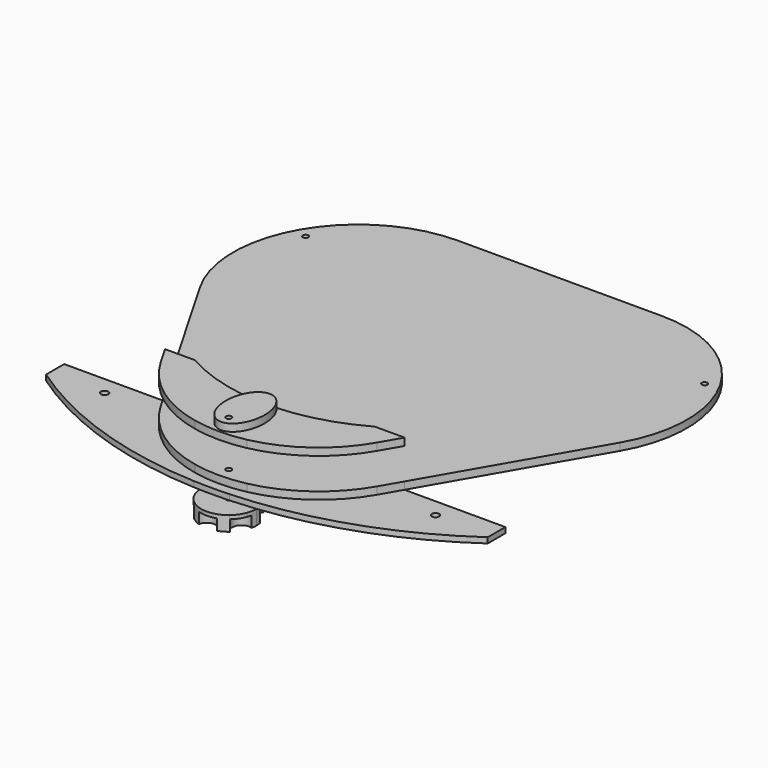
from build123d import *

# Parameters (mm, degrees)
F0_R     = 1.5
F1_DEPTH = 4
F0_R_2   = 2
F2_DEPTH = 3
F3_START = -10
F3_DEPTH = 8
F4_R     = 1.5
F5_DEPTH = 6
F6_START = 21
F6_DEPTH = 4
F7_R     = 1.5
F8_DEPTH = 4


with BuildPart() as f1:
    # F0 (on Top) → F1 (new body)
    with BuildSketch(Plane.XY):
        with BuildLine():
            ThreePointArc((14.9999983029, -125.2980828285), (-2.6585899749, -110.535565822), (-14.0575894796, -130.5310767839))
            ThreePointArc((-14.0575894796, -130.5310767839), (-1.8826e-06, -132), (14.0575857957, -130.5310775623))
            ThreePointArc((14.0575857957, -130.5310775623), (14.7625152359, -127.9566715151), (14.9999983029, -125.2980828285))
        make_face()
        with Locations((-1.6971e-06, -125.2980828285)):
            Circle(F0_R, mode=Mode.SUBTRACT)
        with BuildLine():
            Line((-48.9863926684, -87.1798906476), (-65.1367205046, -87.1798906476))
            Line((-65.1367205046, -87.1798906476), (-58.8897274573, -98))
            ThreePointArc((-58.8897274573, -98), (-39.9361427939, -119.0373009762), (-14.0575894796, -130.5310767839))
            ThreePointArc((-14.0575894796, -130.5310767839), (-2.6585899749, -110.535565822), (14.9999983029, -125.2980828285))
            ThreePointArc((14.9999983029, -125.2980828285), (14.7625152359, -127.9566715151), (14.0575857957, -130.5310775623))
            ThreePointArc((14.0575857957, -130.5310775623), (39.9361412701, -119.0373020819), (58.8897274573, -98))
            Line((58.8897274573, -98), (65.1367205046, -87.1798906476))
            Line((65.1367205046, -87.1798906476), (48.9863926684, -87.1798906476))
            ThreePointArc((48.9863926684, -87.1798906476), (0, -100), (-48.9863926684, -87.1798906476))
        make_face()
        with BuildLine():
            Line((-114.3153532995, -2), (-86.6025397374, -50.0000011103))
            ThreePointArc((-86.6025397374, -50.0000011103), (-86.6025407137, 49.9999994193), (-5.89e-08, 100))
            Line((-5.89e-08, 100), (-55.4256258422, 100))
            ThreePointArc((-55.4256258422, 100), (-114.3153532995, 66), (-114.3153532995, -2))
        make_face()
        with Locations((-108.5113219264, 62.649042884)):
            Circle(F0_R, mode=Mode.SUBTRACT)
        with BuildLine():
            Line((55.4256258422, 100), (-5.89e-08, 100))
            ThreePointArc((-5.89e-08, 100), (70.7106780978, 70.7106781395), (100, 0))
            ThreePointArc((100, 0), (96.5925823782, -25.881905446), (86.6025394097, -50.0000016779))
            Line((86.6025394097, -50.0000016779), (114.3153532995, -2))
            ThreePointArc((114.3153532995, -2), (114.3153532995, 66), (55.4256258422, 100))
        make_face()
        with Locations((108.5113236235, 62.6490399445)):
            Circle(F0_R, mode=Mode.SUBTRACT)
        with BuildLine():
            Line((-86.6025397374, -50.0000011103), (-65.1367205046, -87.1798906476))
            Line((-65.1367205046, -87.1798906476), (-48.9863926684, -87.1798906476))
            ThreePointArc((-48.9863926684, -87.1798906476), (-70.2970532401, -71.1218975124), (-86.6025397374, -50.0000011103))
        make_face()
        with BuildLine():
            ThreePointArc((-86.6025397374, -50.0000011103), (-70.2970532401, -71.1218975124), (-48.9863926684, -87.1798906476))
            Line((-48.9863926684, -87.1798906476), (48.9863926684, -87.1798906476))
            ThreePointArc((48.9863926684, -87.1798906476), (70.2970530071, -71.1218977427), (86.6025394097, -50.0000016779))
            ThreePointArc((86.6025394097, -50.0000016779), (96.5925823782, -25.881905446), (100, 0))
            ThreePointArc((100, 0), (70.7106780978, 70.7106781395), (-5.89e-08, 100))
            ThreePointArc((-5.89e-08, 100), (-86.6025407137, 49.9999994193), (-86.6025397374, -50.0000011103))
        make_face()
        with BuildLine():
            Line((48.9863926684, -87.1798906476), (-48.9863926684, -87.1798906476))
            ThreePointArc((-48.9863926684, -87.1798906476), (0, -100), (48.9863926684, -87.1798906476))
        make_face()
        with BuildLine():
            ThreePointArc((86.6025394097, -50.0000016779), (70.2970530071, -71.1218977427), (48.9863926684, -87.1798906476))
            Line((48.9863926684, -87.1798906476), (65.1367205046, -87.1798906476))
            Line((65.1367205046, -87.1798906476), (86.6025394097, -50.0000016779))
        make_face()
    extrude(amount=F1_DEPTH)


with BuildPart() as f2:
    # F0 (on Top) → F2 (new body)
    with BuildSketch(Plane.XY):
        with BuildLine():
            Line((-65.1367205046, -87.1798906476), (-120.0000016971, -87.1798906476))
            Line((-120.0000016971, -87.1798906476), (-120.0000016971, -99.5014946908))
            ThreePointArc((-120.0000016971, -99.5014946908), (-67.4578593153, -125.9504598013), (-9.6413594448, -136.7891324229))
            ThreePointArc((-9.6413594448, -136.7891324229), (-12.2556461072, -133.946734752), (-14.0575894796, -130.5310767839))
            ThreePointArc((-14.0575894796, -130.5310767839), (-39.9361427939, -119.0373009762), (-58.8897274573, -98))
            Line((-58.8897274573, -98), (-65.1367205046, -87.1798906476))
        make_face()
        with Locations((-90.0000016971, -97.1798906476)):
            Circle(F0_R_2, mode=Mode.SUBTRACT)
        with BuildLine():
            Line((-48.9863926684, -87.1798906476), (-65.1367205046, -87.1798906476))
            Line((-65.1367205046, -87.1798906476), (-58.8897274573, -98))
            ThreePointArc((-58.8897274573, -98), (-39.9361427939, -119.0373009762), (-14.0575894796, -130.5310767839))
            ThreePointArc((-14.0575894796, -130.5310767839), (-2.6585899749, -110.535565822), (14.9999983029, -125.2980828285))
            ThreePointArc((14.9999983029, -125.2980828285), (14.7625152359, -127.9566715151), (14.0575857957, -130.5310775623))
            ThreePointArc((14.0575857957, -130.5310775623), (39.9361412701, -119.0373020819), (58.8897274573, -98))
            Line((58.8897274573, -98), (65.1367205046, -87.1798906476))
            Line((65.1367205046, -87.1798906476), (48.9863926684, -87.1798906476))
            ThreePointArc((48.9863926684, -87.1798906476), (0, -100), (-48.9863926684, -87.1798906476))
        make_face()
        with BuildLine():
            ThreePointArc((14.9999983029, -125.2980828285), (-2.6585899749, -110.535565822), (-14.0575894796, -130.5310767839))
            ThreePointArc((-14.0575894796, -130.5310767839), (-1.8826e-06, -132), (14.0575857957, -130.5310775623))
            ThreePointArc((14.0575857957, -130.5310775623), (14.7625152359, -127.9566715151), (14.9999983029, -125.2980828285))
        make_face()
        with Locations((-1.6971e-06, -125.2980828285)):
            Circle(F0_R, mode=Mode.SUBTRACT)
        with BuildLine():
            ThreePointArc((14.0575857957, -130.5310775623), (12.2659714734, -133.9320797119), (9.6687990395, -136.7660509273))
            ThreePointArc((9.6687990395, -136.7660509273), (67.4950168504, -125.7769999545), (119.9999983029, -99.1714059888))
            Line((119.9999983029, -99.1714059888), (119.9999983029, -87.1798906476))
            Line((119.9999983029, -87.1798906476), (65.1367205046, -87.1798906476))
            Line((65.1367205046, -87.1798906476), (58.8897274573, -98))
            ThreePointArc((58.8897274573, -98), (39.9361412701, -119.0373020819), (14.0575857957, -130.5310775623))
        make_face()
        with Locations((89.9999983029, -97.1798906476)):
            Circle(F0_R_2, mode=Mode.SUBTRACT)
        with BuildLine():
            Line((48.9863926684, -87.1798906476), (-48.9863926684, -87.1798906476))
            ThreePointArc((-48.9863926684, -87.1798906476), (0, -100), (48.9863926684, -87.1798906476))
        make_face()
        with BuildLine():
            ThreePointArc((-14.0575894796, -130.5310767839), (-12.2556461072, -133.946734752), (-9.6413594448, -136.7891324229))
            ThreePointArc((-9.6413594448, -136.7891324229), (0.0139852399, -136.9996629548), (9.6687990395, -136.7660509273))
            ThreePointArc((9.6687990395, -136.7660509273), (12.2659714734, -133.9320797119), (14.0575857957, -130.5310775623))
            ThreePointArc((14.0575857957, -130.5310775623), (-1.8826e-06, -132), (-14.0575894796, -130.5310767839))
        make_face()
    extrude(amount=-F2_DEPTH)


with BuildPart() as f3:
    # F0 (on Top) → F3 (new body)
    with BuildSketch(Plane.XY.offset(F3_START)):
        with BuildLine():
            ThreePointArc((14.9999983029, -125.2980828285), (-2.6585899749, -110.535565822), (-14.0575894796, -130.5310767839))
            ThreePointArc((-14.0575894796, -130.5310767839), (-1.8826e-06, -132), (14.0575857957, -130.5310775623))
            ThreePointArc((14.0575857957, -130.5310775623), (14.7625152359, -127.9566715151), (14.9999983029, -125.2980828285))
        make_face()
        with Locations((-1.6971e-06, -125.2980828285)):
            Circle(F0_R, mode=Mode.SUBTRACT)
        with BuildLine():
            ThreePointArc((-14.0575894796, -130.5310767839), (-12.2556461072, -133.946734752), (-9.6413594448, -136.7891324229))
            ThreePointArc((-9.6413594448, -136.7891324229), (0.0139852399, -136.9996629548), (9.6687990395, -136.7660509273))
            ThreePointArc((9.6687990395, -136.7660509273), (12.2659714734, -133.9320797119), (14.0575857957, -130.5310775623))
            ThreePointArc((14.0575857957, -130.5310775623), (-1.8826e-06, -132), (-14.0575894796, -130.5310767839))
        make_face()
        with BuildLine():
            ThreePointArc((9.6687990395, -136.7660509273), (0.0139852399, -136.9996629548), (-9.6413594448, -136.7891324229))
            ThreePointArc((-9.6413594448, -136.7891324229), (0.0179278392, -140.2980721129), (9.6687990395, -136.7660509273))
        make_face()
    extrude(amount=-F3_DEPTH)

    # F4 (on face) → F5 (cut)
    with BuildSketch(Plane(origin=(0, 0, -18), x_dir=(1, 0, 0), z_dir=(0, 0, -1))):
        with BuildLine():
            ThreePointArc((4.9300663916, 139.4647489374), (0, 140.2980828285), (-4.9300665802, 139.464750053))
            ThreePointArc((-4.9300665802, 139.464750053), (-5.657e-07, 135.2980828285), (4.9300663916, 139.4647489374))
        make_face()
        with BuildLine():
            ThreePointArc((-14.733727842, 128.1118550097), (-12.9903819053, 132.7980842982), (-9.80366039, 136.6509800902))
            ThreePointArc((-9.80366039, 136.6509800902), (-17.3205086414, 135.2980847882), (-14.733727842, 128.1118550097))
        make_face()
        with BuildLine():
            ThreePointArc((-7.9903819053, 132.7980842982), (-8.4663567298, 134.9272146868), (-9.80366039, 136.6509800902))
            ThreePointArc((-9.80366039, 136.6509800902), (-12.9903819053, 132.7980842982), (-14.733727842, 128.1118550097))
            ThreePointArc((-14.733727842, 128.1118550097), (-10.1370268348, 128.6921903832), (-7.9903819053, 132.7980842982))
        make_face()
        with BuildLine():
            ThreePointArc((14.7337250845, 128.1118516757), (12.9903802082, 132.7980813588), (9.8036595647, 136.6509778718))
            ThreePointArc((9.8036595647, 136.6509778718), (8.6602529064, 130.2980818487), (14.7337250845, 128.1118516757))
        make_face()
        with BuildLine():
            ThreePointArc((17.9903802082, 132.7980813588), (15.1195111087, 137.3221062934), (9.8036595647, 136.6509778718))
            ThreePointArc((9.8036595647, 136.6509778718), (12.9903802082, 132.7980813588), (14.7337250845, 128.1118516757))
            ThreePointArc((14.7337250845, 128.1118516757), (17.0962738004, 129.9447258238), (17.9903802082, 132.7980813588))
        make_face()
        with BuildLine():
            ThreePointArc((-7.9903836024, 117.7980842982), (-10.1370280674, 121.9039778905), (-14.7337284787, 122.4843139813))
            ThreePointArc((-14.7337284787, 122.4843139813), (-12.9903836024, 117.7980842982), (-9.8036629589, 113.9451877852))
            ThreePointArc((-9.8036629589, 113.9451877852), (-8.4663586678, 115.6689533978), (-7.9903836024, 117.7980842982))
        make_face()
        with BuildLine():
            ThreePointArc((9.8036569958, 113.9451855669), (12.9903785111, 117.7980813588), (14.7337244478, 122.4843106474))
            ThreePointArc((14.7337244478, 122.4843106474), (8.6602517751, 120.2980818487), (9.8036569958, 113.9451855669))
        make_face()
        with BuildLine():
            ThreePointArc((4.930063186, 111.1314156041), (-2.8285e-06, 115.2980828285), (-4.9300697858, 111.1314167196))
            ThreePointArc((-4.9300697858, 111.1314167196), (-3.3942e-06, 110.2980828285), (4.930063186, 111.1314156041))
        make_face()
        Polygon((3.4999983029, 123.2773568864), (3.4999983029, 127.3188087707), (-1.6971e-06, 129.3395347128), (-3.5000016971, 127.3188087707), (-3.5000016971, 123.2773568864), (-1.6971e-06, 121.2566309442), align=None)
        with Locations((-1.6971e-06, 125.2980828285)):
            Circle(F4_R, mode=Mode.SUBTRACT)
    extrude(amount=-F5_DEPTH, mode=Mode.SUBTRACT)


with BuildPart() as f6:
    # F0 (on Top) → F6 (new body)
    with BuildSketch(Plane.XY.offset(F6_START)):
        with BuildLine():
            ThreePointArc((14.9999983029, -125.2980828285), (-2.6585899749, -110.535565822), (-14.0575894796, -130.5310767839))
            ThreePointArc((-14.0575894796, -130.5310767839), (-1.8826e-06, -132), (14.0575857957, -130.5310775623))
            ThreePointArc((14.0575857957, -130.5310775623), (14.7625152359, -127.9566715151), (14.9999983029, -125.2980828285))
        make_face()
        with Locations((-1.6971e-06, -125.2980828285)):
            Circle(F0_R, mode=Mode.SUBTRACT)
        with BuildLine():
            Line((-48.9863926684, -87.1798906476), (-65.1367205046, -87.1798906476))
            Line((-65.1367205046, -87.1798906476), (-58.8897274573, -98))
            ThreePointArc((-58.8897274573, -98), (-39.9361427939, -119.0373009762), (-14.0575894796, -130.5310767839))
            ThreePointArc((-14.0575894796, -130.5310767839), (-2.6585899749, -110.535565822), (14.9999983029, -125.2980828285))
            ThreePointArc((14.9999983029, -125.2980828285), (14.7625152359, -127.9566715151), (14.0575857957, -130.5310775623))
            ThreePointArc((14.0575857957, -130.5310775623), (39.9361412701, -119.0373020819), (58.8897274573, -98))
            Line((58.8897274573, -98), (65.1367205046, -87.1798906476))
            Line((65.1367205046, -87.1798906476), (48.9863926684, -87.1798906476))
            ThreePointArc((48.9863926684, -87.1798906476), (0, -100), (-48.9863926684, -87.1798906476))
        make_face()
    extrude(amount=F6_DEPTH)


with BuildPart() as f8:
    # F7 (on face) → F8 (new body)
    with BuildSketch(Plane.XY.offset(25)):
        with BuildLine():
            ThreePointArc((5.4254401673, -99.8527145299), (0, -100), (-5.4254401673, -99.8527145299))
            add(Edge.make_bspline(
                [(-5.4254401673, -99.8527145299), (-38.1652299211, -130.5071302652), (0, -130.5071302652), (38.1652299211, -130.5071302652), (5.4254401673, -99.8527145299)],
                knots=[0.5397379565, 0.5397379565, 0.5397379565, 3.1415926536, 3.1415926536, 5.7434473507, 5.7434473507, 5.7434473507], degree=2, weights=[1, 0.2666051595, 1, 0.2666051595, 1]))
        make_face()
        with Locations((-1.6971e-06, -125.2980828285)):
            Circle(F7_R, mode=Mode.SUBTRACT)
        with BuildLine():
            add(Edge.make_bspline(
                [(5.4254401673, -99.8527145299), (2.920289316, -97.5071302652), (0, -97.5071302652)],
                knots=[5.7434473507, 5.7434473507, 5.7434473507, 6.2831853072, 6.2831853072, 6.2831853072], degree=2, weights=[1, 0.9638058357, 1]))
            add(Edge.make_bspline(
                [(0, -97.5071302652), (-2.920289316, -97.5071302652), (-5.4254401673, -99.8527145299)],
                knots=[0, 0, 0, 0.5397379565, 0.5397379565, 0.5397379565], degree=2, weights=[1, 0.9638058357, 1]))
            ThreePointArc((-5.4254401673, -99.8527145299), (0, -100), (5.4254401673, -99.8527145299))
        make_face()
    extrude(amount=F8_DEPTH)


solid = Compound([f1.part, f2.part, f3.part, f6.part, f8.part])
